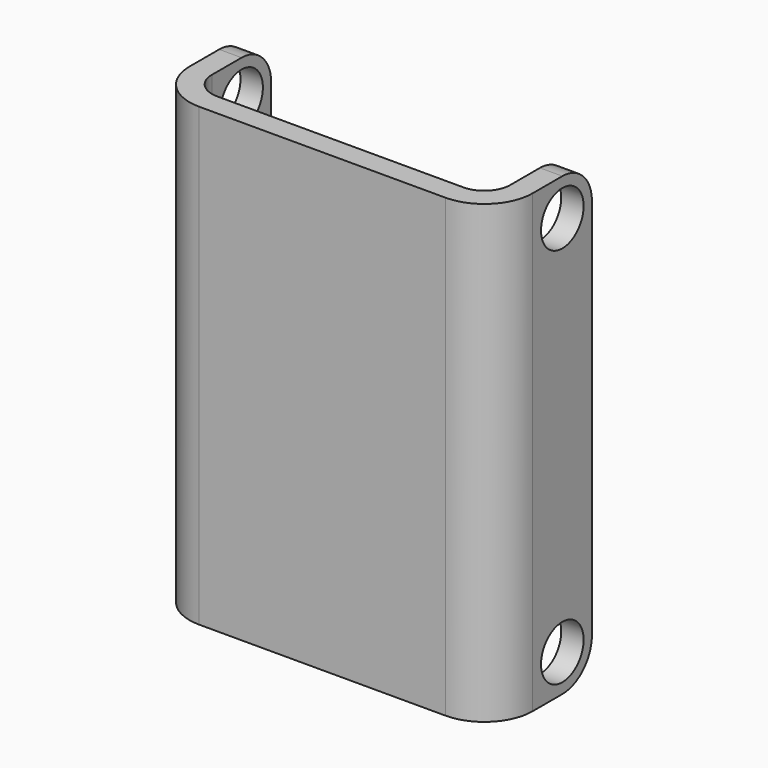
from build123d import *

# Parameters (mm, degrees)
F1_DEPTH = 34.7990414
F2_R     = 3.69316
F3_R     = 1.98374
F4_R     = 2.032
F5_DEPTH = 26.1874
F6_R     = 2.82575


with BuildPart() as f1:
    # F0 (on Top) → F1 (new body)
    with BuildSketch(Plane.XY):
        Polygon((0, 7.63524), (0, 0), (-22.76856, 0), (-22.76856, 7.63524), (-24.47798, 7.63524), (-24.47798, -1.70942), (1.70942, -1.70942), (1.70942, 7.63524), align=None)
    extrude(amount=F1_DEPTH)

    # F2
    f2_edges = [f1.edges().sort_by_distance(p)[0] for p in [
        (1.70942, -1.70942, 17.399521),
        (-24.47798, -1.70942, 17.399521),
    ]]
    fillet(f2_edges, radius=F2_R)

    # F3
    f3_edges = [f1.edges().sort_by_distance(p)[0] for p in [
        (0, 0, 17.399521),
        (-22.76856, 0, 17.399521),
    ]]
    fillet(f3_edges, radius=F3_R)

    # F4 (on face) → F5 (cut, through all)
    with BuildSketch(Plane.YZ.offset(1.70942)):
        with Locations((4.80949, 2.82575)):
            Circle(F4_R)
        with Locations((4.80949, 31.9732914)):
            Circle(F4_R)
    extrude(amount=-F5_DEPTH, mode=Mode.SUBTRACT)

    # F6
    f6_edges = [f1.edges().sort_by_distance(p)[0] for p in [
        (0.85471, 7.63524, 34.799041),
        (-23.62327, 7.63524, 34.799041),
        (0.85471, 7.63524, 0),
        (-23.62327, 7.63524, 0),
    ]]
    fillet(f6_edges, radius=F6_R)


solid = f1.part
